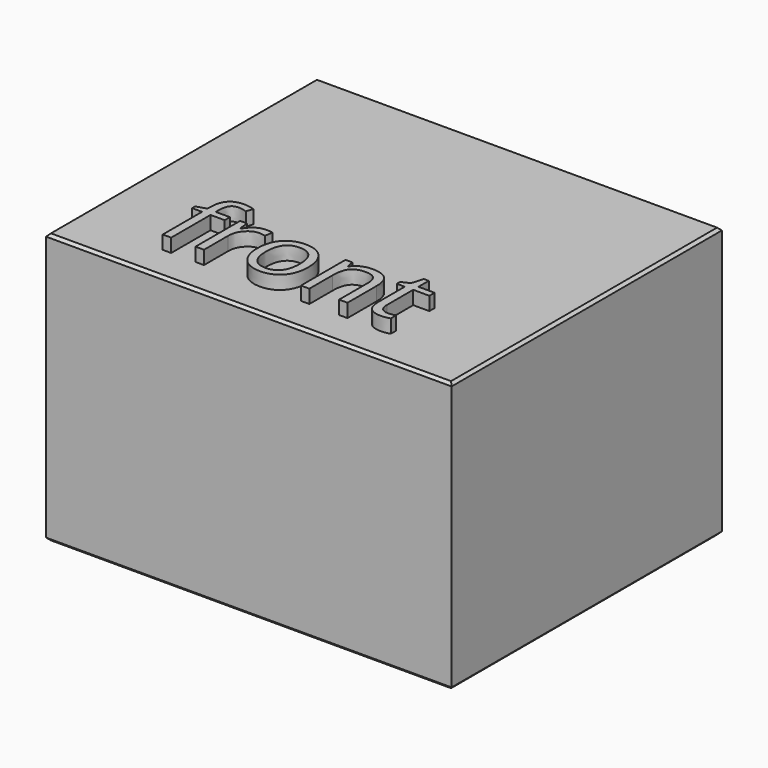
from build123d import *

# Parameters (mm, degrees)
F0_W         = 30
F0_H         = 25
F1_DEPTH     = 20
F2_SIZE      = 0.2
F3_TEXT_SIZE = 7.7019743104
F4_DEPTH     = 1


# Not quite as in the source:
# - Text() gives the source's letters only with a copy of the font that has no kerning and outlines rounded to 1/6400 em; it was checked with that copy


with BuildPart() as f1:
    # F0 (on Top) → F1 (new body)
    with BuildSketch(Plane.XY):
        Rectangle(F0_W, F0_H)
    extrude(amount=F1_DEPTH)

    # F2
    f2_edges = [f1.edges().sort_by_distance(p)[0] for p in [
        (0, -12.5, 20),
        (-15, 0, 20),
        (0, 12.5, 20),
        (15, 0, 20),
        (0, -12.5, 0),
        (-15, 0, 0),
        (0, 12.5, 0),
        (15, 0, 0),
    ]]
    chamfer(f2_edges, length=F2_SIZE)

    # F3 (on face) → F4 (join)
    with BuildSketch(Plane.XY.offset(20)):
        with Locations((-9.3109775335, -9.8809525371)):
            Text('front', F3_TEXT_SIZE, font='Open Sans', text_align=(TextAlign.LEFT, TextAlign.BOTTOM))
    extrude(amount=F4_DEPTH)


solid = f1.part
